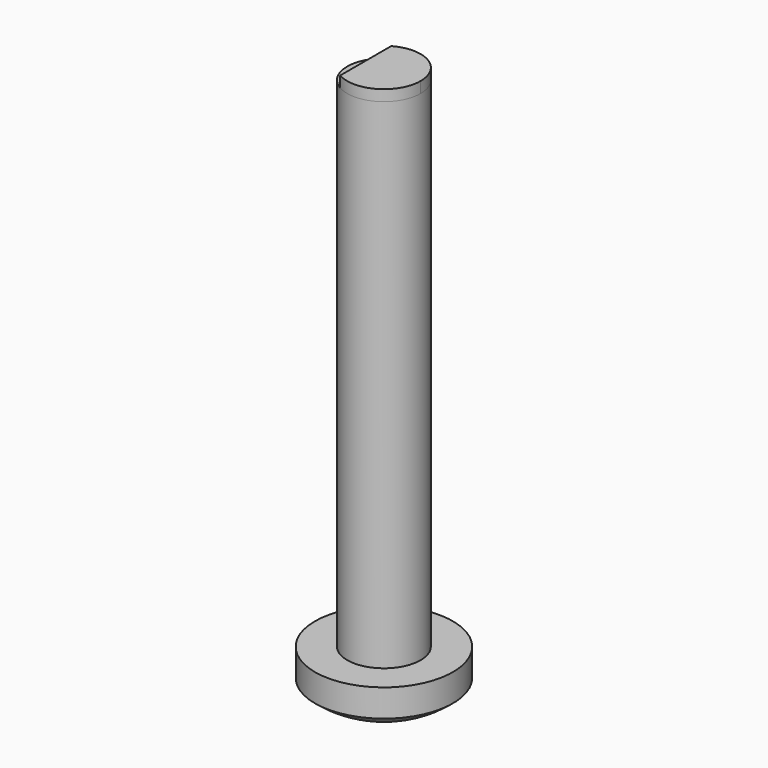
from build123d import *

# Parameters (mm, degrees)
F0_W     = 1.27
F0_H     = 17.272
F3_DEPTH = 0.381


# Not quite as in the source:
# - a feature names something its author has since deleted; it is built from what else it names


with BuildPart() as f1:
    # F0 (on Front) → F1 (revolve)
    with BuildSketch(Plane.XZ):
        with Locations((-38.810752406, 44.918222718)):
            Rectangle(F0_W, F0_H)
        with BuildLine():
            Line((-38.175752406, 36.282222718), (-39.445752406, 36.282222718))
            Line((-39.445752406, 36.282222718), (-40.563352406, 36.282222718))
            Line((-40.563352406, 36.282222718), (-40.563352406, 35.9659250826))
            Line((-40.563352406, 35.9659250826), (-40.563352406, 35.329721868))
            ThreePointArc((-40.563352406, 35.329721868), (-39.5245363872, 34.7150900066), (-38.3366011083, 34.5012657344))
            Line((-38.3366011083, 34.5012657344), (-38.175752406, 34.5012657344))
            Line((-38.175752406, 34.5012657344), (-38.175752406, 35.1264222169))
            Line((-38.175752406, 35.1264222169), (-38.175752406, 36.282222718))
        make_face()
    revolve(axis=Axis((-38.175752406, 0, 44.918222718), (0, 0, -1)))

    # F2 (on face) → F3 (join)
    with BuildSketch(Plane.XY.offset(53.554222718)):
        with BuildLine():
            Line((-38.8069041073, 1.1020651206), (-38.8069041073, 0))
            Line((-38.8069041073, 0), (-38.8069041073, -1.1020651206))
            ThreePointArc((-38.8069041073, -1.1020651206), (-37.5388311631, -1.0987407931), (-36.905752406, 0))
            ThreePointArc((-36.905752406, 0), (-37.5388311631, 1.0987407931), (-38.8069041073, 1.1020651206))
        make_face()
    extrude(amount=F3_DEPTH)


solid = f1.part
